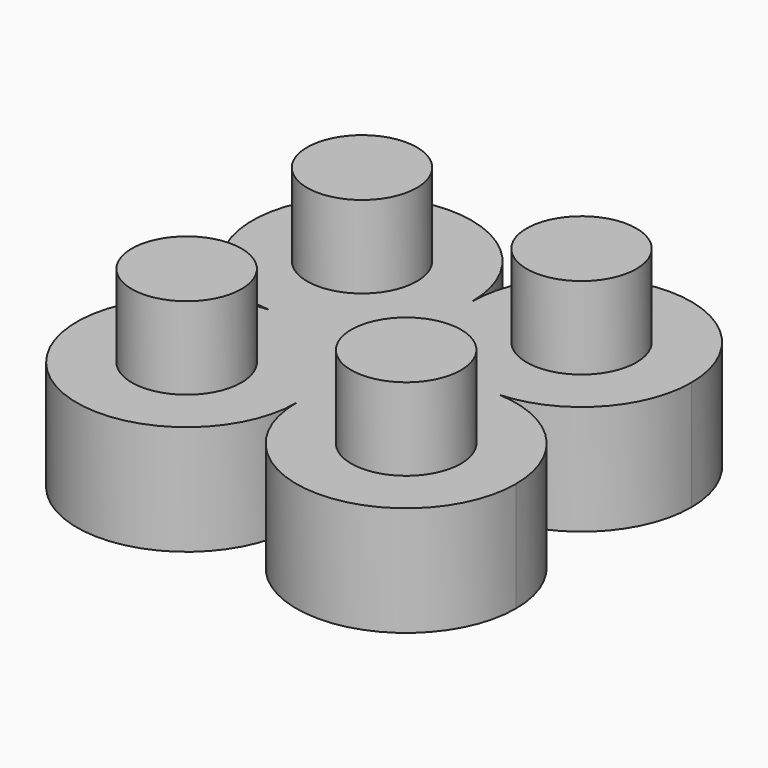
from build123d import *

# Parameters (mm, degrees)
F0_R     = 1
F1_DEPTH = 3.5
F2_DEPTH = 2
F3_DEPTH = 2


with BuildPart() as f1:
    # F0 (on Top) → F1 (new body)
    with BuildSketch(Plane.XY):
        with Locations((-2.3999998812, 1.8953582125)):
            Circle(F0_R)
    extrude(amount=F1_DEPTH)



with BuildPart() as f1b:
    # F0 (on Top) → F1, piece 2 (new body)
    with BuildSketch(Plane.XY):
        with Locations((1.6000001188, 1.8953582125)):
            Circle(F0_R)
    extrude(amount=F1_DEPTH)


with BuildPart() as f1c:
    # F0 (on Top) → F1, piece 3 (new body)
    with BuildSketch(Plane.XY):
        with Locations((1.6000001188, -2.0999999251)):
            Circle(F0_R)
    extrude(amount=F1_DEPTH)


with BuildPart() as f1d:
    # F0 (on Top) → F1, piece 4 (new body)
    with BuildSketch(Plane.XY):
        with Locations((-2.3999998812, -2.0999999251)):
            Circle(F0_R)
    extrude(amount=F1_DEPTH)


with BuildPart() as f1_1:
    add(f1.part)

    add(f1d.part)  # F2 merges F1d
    # F0 (on Top) → F2 (join)
    with BuildSketch(Plane.XY):
        with BuildLine():
            ThreePointArc((-2.4963240114, -0.1023208563), (-3.7797374902, -3.5478687487), (-0.3999998812, -2.0999999251))
            ThreePointArc((-0.3999998812, -2.0999999251), (-0.9521310576, -0.7202623161), (-2.3036757509, -0.1023208563))
            ThreePointArc((-2.3036757509, -0.1023208563), (-2.3999998812, -0.1046417875), (-2.4963240114, -0.1023208563))
        make_face()
        with Locations((-2.3999998812, -2.0999999251)):
            Circle(F0_R, mode=Mode.SUBTRACT)
        with BuildLine():
            ThreePointArc((-2.4963240114, -0.1023208563), (-2.3999998812, -0.1046417875), (-2.3036757509, -0.1023208563))
            ThreePointArc((-2.3036757509, -0.1023208563), (-2.3999998812, -0.0999999251), (-2.4963240114, -0.1023208563))
        make_face()
        with BuildLine():
            ThreePointArc((-2.4963240114, -0.1023208563), (-2.3999998812, -0.0999999251), (-2.3036757509, -0.1023208563))
            ThreePointArc((-2.3036757509, -0.1023208563), (-0.9521310576, 0.5156206035), (-0.3999998812, 1.8953582125))
            ThreePointArc((-0.3999998812, 1.8953582125), (-3.7797374902, 3.343227036), (-2.4963240114, -0.1023208563))
        make_face()
        with Locations((-2.3999998812, 1.8953582125)):
            Circle(F0_R, mode=Mode.SUBTRACT)
    extrude(amount=F2_DEPTH)


    add(f1b.part)  # F2#2 merges F1b

    add(f1c.part)  # F2#2 merges F1c
    # F0 (on Top) → F2, piece 2 (join)
    with BuildSketch(Plane.XY):
        with BuildLine():
            ThreePointArc((1.5036759886, -0.1023208563), (0.1521312953, -0.7202623161), (-0.3999998812, -2.0999999251))
            ThreePointArc((-0.3999998812, -2.0999999251), (1.6000001188, -4.0999999251), (3.6000001188, -2.0999999251))
            ThreePointArc((3.6000001188, -2.0999999251), (3.0478689424, -0.7202623161), (1.6963242491, -0.1023208563))
            ThreePointArc((1.6963242491, -0.1023208563), (1.6000001188, -0.1046417875), (1.5036759886, -0.1023208563))
        make_face()
        with Locations((1.6000001188, -2.0999999251)):
            Circle(F0_R, mode=Mode.SUBTRACT)
        with BuildLine():
            ThreePointArc((-0.3999998812, 1.8953582125), (0.1521312953, 0.5156206035), (1.5036759886, -0.1023208563))
            ThreePointArc((1.5036759886, -0.1023208563), (1.6000001188, -0.0999999251), (1.6963242491, -0.1023208563))
            ThreePointArc((1.6963242491, -0.1023208563), (3.0478689424, 0.5156206035), (3.6000001188, 1.8953582125))
            ThreePointArc((3.6000001188, 1.8953582125), (1.6000001188, 3.8953582125), (-0.3999998812, 1.8953582125))
        make_face()
        with Locations((1.6000001188, 1.8953582125)):
            Circle(F0_R, mode=Mode.SUBTRACT)
        with BuildLine():
            ThreePointArc((1.6963242491, -0.1023208563), (1.6000001188, -0.0999999251), (1.5036759886, -0.1023208563))
            ThreePointArc((1.5036759886, -0.1023208563), (1.6000001188, -0.1046417875), (1.6963242491, -0.1023208563))
        make_face()
    extrude(amount=F2_DEPTH)

    # F0 (on Top) → F3 (join)
    with BuildSketch(Plane.XY):
        with BuildLine():
            ThreePointArc((-2.3036757509, -0.1023208563), (-0.9521310576, -0.7202623161), (-0.3999998812, -2.0999999251))
            ThreePointArc((-0.3999998812, -2.0999999251), (0.1521312953, -0.7202623161), (1.5036759886, -0.1023208563))
            ThreePointArc((1.5036759886, -0.1023208563), (0.1521312953, 0.5156206035), (-0.3999998812, 1.8953582125))
            ThreePointArc((-0.3999998812, 1.8953582125), (-0.9521310576, 0.5156206035), (-2.3036757509, -0.1023208563))
        make_face()
    extrude(amount=F3_DEPTH)


solid = f1_1.part
